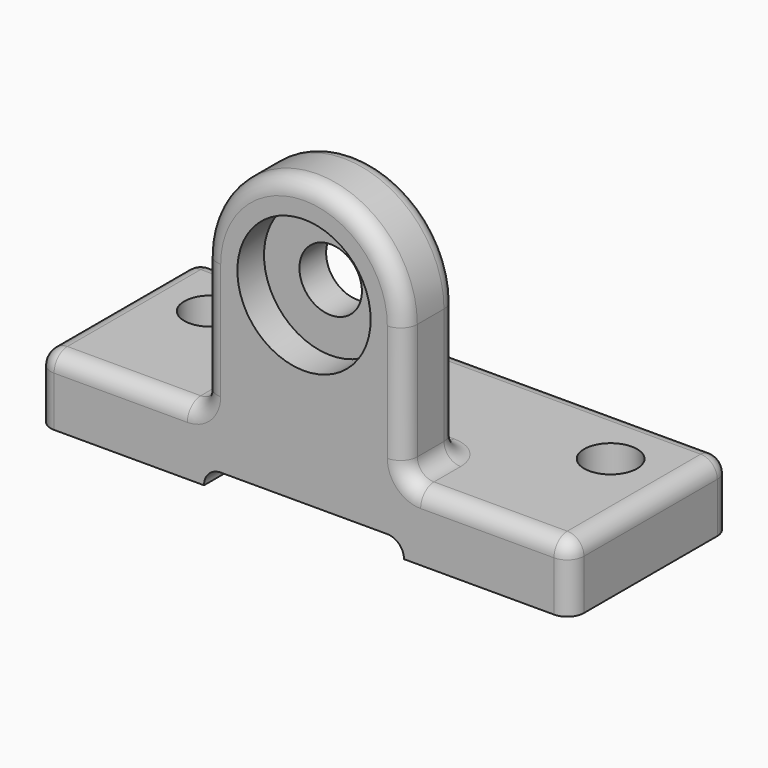
from build123d import *

# Parameters (mm, degrees)
F0_W           = 101.6
F0_H           = 38.1
F1_DEPTH       = 12.7
F2_W           = 38.1
F2_H           = 12.7
F3_DEPTH       = 12.7
F4_D           = 11.90625
F4_CBORE_D     = 25.4
F4_CBORE_DEPTH = 6.35
F5_W           = 38.1
F5_H           = 3.175
F6_DEPTH       = 38.101
F8_D           = 10.0838
F9_R           = 3.17499
F10_R          = 3.17499


# Not quite as in the source:
# - a fillet or chamfer is up to 0.001 mm smaller than in the source, because OpenCascade refuses the exact size
# - a length typed as a fraction of an inch, garbled in the dataset ("3 / 203.2 mm" for 3/8 in), is restored


with BuildPart() as f1:
    # F0 (on Top) → F1 (new body)
    with BuildSketch(Plane.XY):
        with Locations((50.8, 19.05)):
            Rectangle(F0_W, F0_H)
    extrude(amount=F1_DEPTH)

    # F2 (on face) → F3 (join)
    with BuildSketch(Plane.XZ):
        with BuildLine():
            Line((31.75, 38.1), (31.75, 12.7))
            Line((31.75, 12.7), (69.85, 12.7))
            Line((69.85, 12.7), (69.85, 38.1))
            ThreePointArc((69.85, 38.1), (50.8, 57.15), (31.75, 38.1))
        make_face()
        with Locations((50.8, 6.35)):
            Rectangle(F2_W, F2_H)
    extrude(amount=-F3_DEPTH)

    # F4 (through all)
    with Locations(Plane.XZ):
        with Locations((50.8, 38.1)):
            CounterBoreHole(F4_D / 2, F4_CBORE_D / 2, F4_CBORE_DEPTH)

    # F5 (on face) → F6 (cut, through all)
    with BuildSketch(Plane(origin=(0, 38.1, 0), x_dir=(-1, 0, 0), z_dir=(0, 1, 0))):
        with Locations((-50.7999828577, 1.5875)):
            Rectangle(F5_W, F5_H)
    extrude(amount=-F6_DEPTH, mode=Mode.SUBTRACT)

    # F8 (through all)
    with Locations(Plane.XY.offset(12.7)):
        with Locations((12.7, 25.4), (88.9, 25.4)):
            Hole(F8_D / 2)

    # F9 (radius 3.175 in the source; OpenCascade refuses exactly that, so slightly less here)
    f9_edges = [f1.edges().sort_by_distance(p)[0] for p in [
        (0, 0, 6.35),
        (101.6, 0, 6.35),
        (101.6, 38.1, 6.35),
        (0, 38.1, 6.35),
        (31.749983, 19.05, 3.175),
        (69.849983, 19.05, 3.175),
    ]]
    fillet(f9_edges, radius=F9_R)

    # F10 (radius 3.175 in the source; OpenCascade refuses exactly that, so slightly less here)
    f10_edges = [f1.edges().sort_by_distance(p)[0] for p in [
        (50.8, 0, 57.15),
        (50.8, 12.7, 57.15),
        (31.75, 0, 25.4),
        (69.85, 0, 25.4),
        (31.75, 12.7, 25.4),
        (17.462495, 0, 12.7),
        (0.929933, 0.929933, 12.7),
        (0, 19.05, 12.7),
        (0.929933, 37.170067, 12.7),
        (50.8, 38.1, 12.7),
        (100.670067, 37.170067, 12.7),
        (101.6, 19.05, 12.7),
        (100.670067, 0.929933, 12.7),
        (84.137505, 0, 12.7),
        (50.8, 12.7, 12.7),
        (31.75, 6.35, 12.7),
        (69.85, 12.7, 25.4),
        (69.85, 6.35, 12.7),
    ]]
    fillet(f10_edges, radius=F10_R)


solid = f1.part
